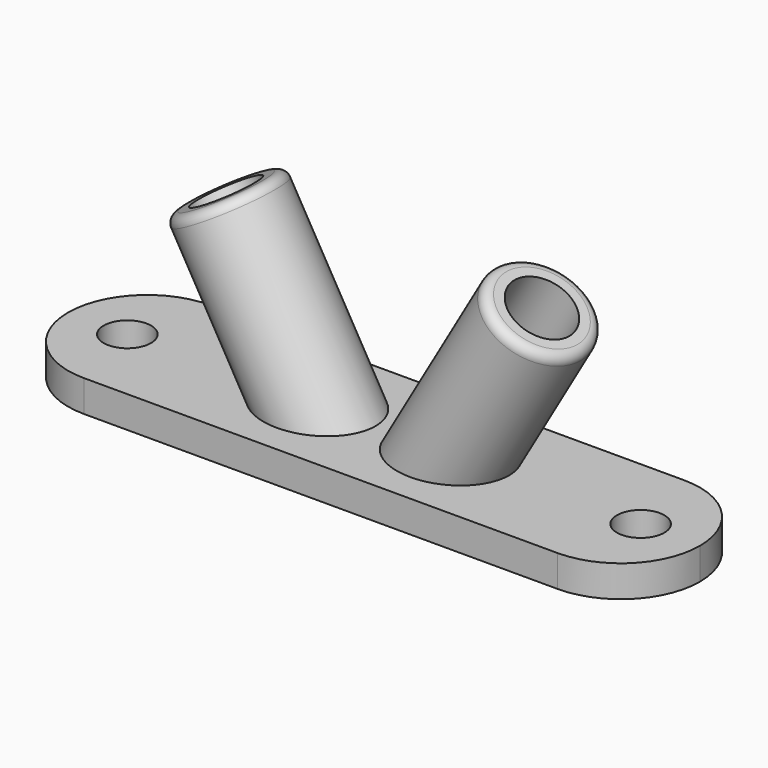
from build123d import *

# Parameters (mm, degrees)
F0_W      = 40
F0_H      = 10
F0_R      = 1.5
F1_DEPTH  = 2
F7_R      = 3.2
F7_R_2    = 2
F9_R      = 3.2
F9_R_2    = 2
F11_R     = 4.99999
F12_DEPTH = 2.001
F13_DEPTH = 2.0010001
F14_R     = 0.6


# Not quite as in the source:
# - a fillet or chamfer is up to 0.001 mm smaller than in the source, because OpenCascade refuses the exact size


with BuildPart() as f1:
    # F0 (on Top) → F1 (new body)
    with BuildSketch(Plane.XY):
        Rectangle(F0_W, F0_H)
        with Locations((-16.25, 0)):
            Circle(F0_R, mode=Mode.SUBTRACT)
        with Locations((16.25, 0)):
            Circle(F0_R, mode=Mode.SUBTRACT)
    extrude(amount=F1_DEPTH)

    # F7 (on line) → F8 (join, up to the next surface of F1)
    with BuildSketch(Plane(origin=(7.6961524227, 0, 13.3301270189), x_dir=(0.8660254038, 0, -0.5), z_dir=(-0.5, 0, -0.8660254038))):
        with Locations((2.6602540378, 0)):
            Circle(F7_R)
        with Locations((2.6602540378, 0)):
            Circle(F7_R_2, mode=Mode.SUBTRACT)
    extrude(until=Until.NEXT)

    # F9 (on line) → F10 (join, up to the next surface of F1)
    with BuildSketch(Plane(origin=(-7.6961524227, 0, 13.3301270189), x_dir=(0.8660254038, 0, 0.5), z_dir=(0.5, 0, -0.8660254038))):
        with Locations((-2.6602540378, 0)):
            Circle(F9_R)
        with Locations((-2.6602540378, 0)):
            Circle(F9_R_2, mode=Mode.SUBTRACT)
    extrude(until=Until.NEXT)

    # F11 (radius 5 in the source; OpenCascade refuses exactly that, so slightly less here)
    f11_edges = [f1.edges().sort_by_distance(p)[0] for p in [
        (-20, -5, 1),
        (20, -5, 1),
        (20, 5, 1),
        (-20, 5, 1),
    ]]
    fillet(f11_edges, radius=F11_R)

    # F12 (cut, through all): a face of the model
    f12_faces = [f1.faces().sort_by_distance(p)[0] for p in [
        (-4.2264973081, 0, 2),
    ]]
    extrude(f12_faces, amount=-F12_DEPTH, mode=Mode.SUBTRACT)

    # F13 (cut, through all): a face of the model
    f13_faces = [f1.faces().sort_by_distance(p)[0] for p in [
        (4.2264973081, 0, 2),
    ]]
    extrude(f13_faces, amount=-F13_DEPTH, mode=Mode.SUBTRACT)

    # F14
    f14_edges = [f1.edges().sort_by_distance(p)[0] for p in [
        (-12.771281, 0, 10.4),
        (7.228719, 0, 13.6),
    ]]
    fillet(f14_edges, radius=F14_R)


solid = f1.part
